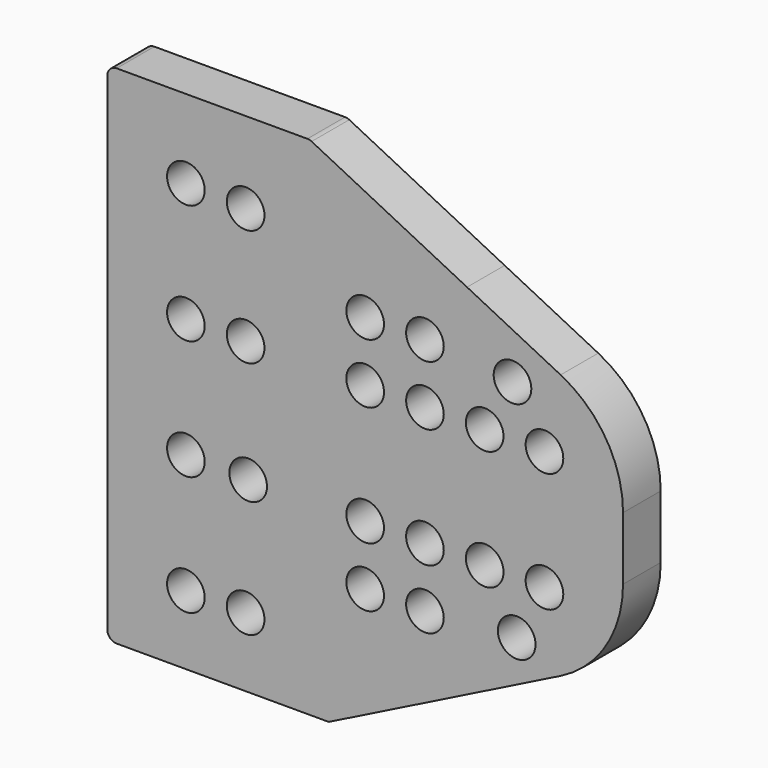
from build123d import *

# Parameters (mm, degrees)
F0_R     = 0.4
F0_W     = 4.21
F0_H     = 2.54
F1_DEPTH = 1


# Not quite as in the source:
# - ends of sketch curves that miss each other by under 0.0002 mm in the source are joined


with BuildPart() as f1:
    # F0 (on Front) → F1 (new body)
    with BuildSketch(Plane.XZ):
        with BuildLine():
            Line((4.153313, 2.713934), (2.1644269248, 3.7083768497))
            Line((2.1644269248, 3.7083768497), (-0.77, 3.708377))
            ThreePointArc((-0.77, 3.708377), (-1.1235533906, 3.5619303906), (-1.27, 3.208377))
            Line((-1.27, 3.208377), (-1.27, 2.438377))
            Line((-1.27, 2.438377), (-1.27, -0.101623))
            Line((-1.27, -0.101623), (5.48, -0.101623))
            Line((5.48, -0.101623), (5.48, 0.567309))
            ThreePointArc((5.48, 0.567309), (5.1215620576, 1.8290634789), (4.153313, 2.713934))
        make_face()
        with Locations((0, 1.168377)):
            Circle(F0_R, mode=Mode.SUBTRACT)
        with Locations((1.27, 1.168377)):
            Circle(F0_R, mode=Mode.SUBTRACT)
        with Locations((2.54, 1.168377)):
            Circle(F0_R, mode=Mode.SUBTRACT)
        with Locations((0, 2.438377)):
            Circle(F0_R, mode=Mode.SUBTRACT)
        with Locations((1.27, 2.438377)):
            Circle(F0_R, mode=Mode.SUBTRACT)
        with Locations((3.81, 1.168377)):
            Circle(F0_R, mode=Mode.SUBTRACT)
        with Locations((3.130691, 2.25)):
            Circle(F0_R, mode=Mode.SUBTRACT)
        with BuildLine():
            Line((2.1644269248, 3.7083768497), (-1.13809, 5.359635))
            ThreePointArc((-1.13809, 5.359635), (-1.1815821983, 5.3753997465), (-1.227533, 5.38075))
            Line((-1.227533, 5.38075), (-5.28, 5.38075))
            ThreePointArc((-5.28, 5.38075), (-5.4214213562, 5.3221713562), (-5.48, 5.18075))
            Line((-5.48, 5.18075), (-5.48, 2.438377))
            Line((-5.48, 2.438377), (-1.27, 2.438377))
            Line((-1.27, 2.438377), (-1.27, 3.208377))
            ThreePointArc((-1.27, 3.208377), (-1.1235533906, 3.5619303906), (-0.77, 3.708377))
            Line((-0.77, 3.708377), (2.1644269248, 3.7083768497))
        make_face()
        with Locations((-3.81, 3.708377)):
            Circle(F0_R, mode=Mode.SUBTRACT)
        with Locations((-2.54, 3.65085)):
            Circle(F0_R, mode=Mode.SUBTRACT)
        with Locations((-3.375, 1.168377)):
            Rectangle(F0_W, F0_H)
        with Locations((-3.81, 1.168377)):
            Circle(F0_R, mode=Mode.SUBTRACT)
        with Locations((-2.54, 1.168377)):
            Circle(F0_R, mode=Mode.SUBTRACT)
        with Locations((-3.375, -1.371623)):
            Rectangle(F0_W, F0_H)
        with Locations((-3.81, -1.371623)):
            Circle(F0_R, mode=Mode.SUBTRACT)
        with Locations((-2.486643, -1.406452)):
            Circle(F0_R, mode=Mode.SUBTRACT)
        with BuildLine():
            Line((-1.27, -3.411623), (-1.27, -2.641623))
            Line((-1.27, -2.641623), (-5.48, -2.641623))
            Line((-5.48, -2.641623), (-5.48, -5.18075))
            ThreePointArc((-5.48, -5.18075), (-5.4214213562, -5.3221713562), (-5.28, -5.38075))
            Line((-5.28, -5.38075), (-0.773828, -5.38075))
            Line((-0.773828, -5.38075), (2.1644269193, -3.9116228385))
            Line((2.1644269193, -3.9116228385), (-0.77, -3.911623))
            ThreePointArc((-0.77, -3.911623), (-1.1235533906, -3.7651763906), (-1.27, -3.411623))
        make_face()
        with Locations((-3.81, -3.911623)):
            Circle(F0_R, mode=Mode.SUBTRACT)
        with Locations((-2.54, -3.911623)):
            Circle(F0_R, mode=Mode.SUBTRACT)
        with BuildLine():
            Line((5.48, -0.770555), (5.48, -0.101623))
            Line((5.48, -0.101623), (-1.27, -0.101623))
            Line((-1.27, -0.101623), (-1.27, -2.641623))
            Line((-1.27, -2.641623), (-1.27, -3.411623))
            ThreePointArc((-1.27, -3.411623), (-1.1235533906, -3.7651763906), (-0.77, -3.911623))
            Line((-0.77, -3.911623), (2.164427, -3.911623))
            Line((2.164427, -3.911623), (4.153313, -2.91718))
            ThreePointArc((4.153313, -2.91718), (5.1215620576, -2.0323094789), (5.48, -0.770555))
        make_face()
        with Locations((0, -2.641623)):
            Circle(F0_R, mode=Mode.SUBTRACT)
        with Locations((1.27, -2.641623)):
            Circle(F0_R, mode=Mode.SUBTRACT)
        with Locations((0, -1.371623)):
            Circle(F0_R, mode=Mode.SUBTRACT)
        with Locations((1.27, -1.371623)):
            Circle(F0_R, mode=Mode.SUBTRACT)
        with Locations((2.54, -1.371623)):
            Circle(F0_R, mode=Mode.SUBTRACT)
        with Locations((3.220234, -2.503932)):
            Circle(F0_R, mode=Mode.SUBTRACT)
        with Locations((3.81, -1.371623)):
            Circle(F0_R, mode=Mode.SUBTRACT)
    extrude(amount=F1_DEPTH)


solid = f1.part
